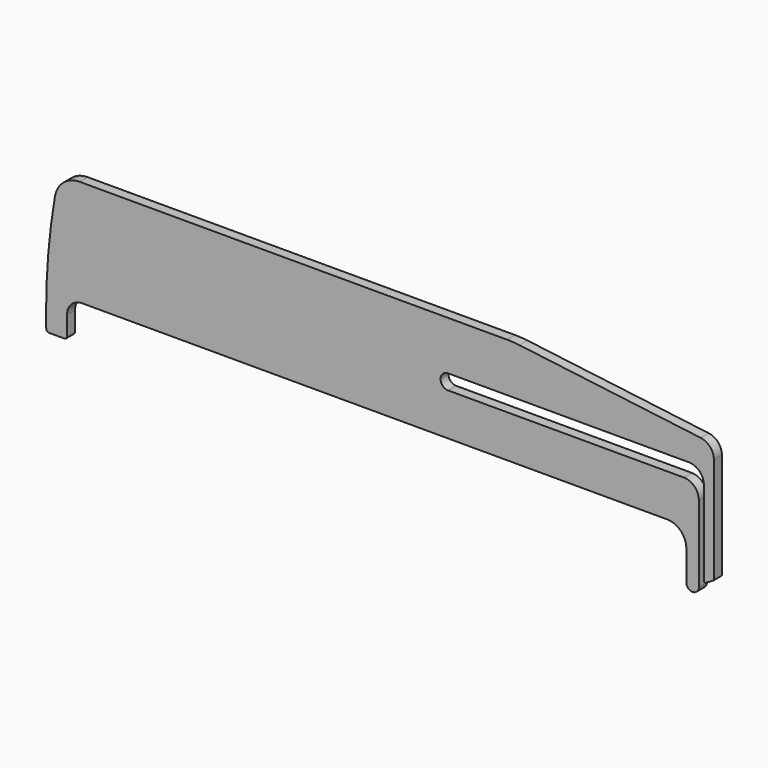
from build123d import *

# Parameters (mm, degrees)
F1_DEPTH = 1


# Not quite as in the source:
# - a feature names something its author has since deleted; it is built from what else it names


with BuildPart() as f1:
    # F0 (on Front) → F1 (new body, symmetric)
    with BuildSketch(Plane.XZ):
        with BuildLine():
            ThreePointArc((-58.215127866, 20.8417536759), (-59.5395660257, 10.4582609311), (-59.9821, 0))
            ThreePointArc((-59.9821, 0), (-59.9729371877, -1.5061942231), (-59.9454501071, -3.0121654896))
            ThreePointArc((-59.9454501071, -3.0121654896), (-59.7948238827, -3.3578286914), (-59.4455981282, -3.5))
            Line((-59.4455981282, -3.5), (-56.3175, -3.5))
            ThreePointArc((-56.3175, -3.5), (-55.9639466094, -3.3535533906), (-55.8175, -3))
            Line((-55.8175, -3), (-55.8175, 0.8354))
            ThreePointArc((-55.8175, 0.8354), (-54.9388203436, 2.9567203436), (-52.8175, 3.8354))
            Line((-52.8175, 3.8354), (63.8175, 3.8354))
            ThreePointArc((63.8175, 3.8354), (66.5295373486, 2.7120373486), (67.6529, 0))
            Line((67.6529, 0), (67.6529, -6))
            ThreePointArc((67.6529, -6), (68.9029, -7.25), (70.1529, -6))
            Line((70.1529, -6), (70.1529, 9.2687909752))
            ThreePointArc((70.1529, 9.2687909752), (69.2742203436, 11.3901113188), (67.1529, 12.2687909752))
            Line((67.1529, 12.2687909752), (20.1529, 12.2687909752))
            ThreePointArc((20.1529, 12.2687909752), (18.6529, 13.7687909752), (20.1529, 15.2687909752))
            Line((20.1529, 15.2687909752), (68.1529, 15.2687909752))
            ThreePointArc((68.1529, 15.2687909752), (70.2742203436, 14.3901113188), (71.1529, 12.2687909752))
            Line((71.1529, 12.2687909752), (71.1529, -4.5669872981))
            ThreePointArc((71.1529, -4.5669872981), (71.2779, -4.7834936491), (71.5279, -4.7834936491))
            Line((71.5279, -4.7834936491), (73.0279, -3.9174682453))
            ThreePointArc((73.0279, -3.9174682453), (73.1194063509, -3.8259618943), (73.1529, -3.7009618943))
            Line((73.1529, -3.7009618943), (73.1529, 17.3516533444))
            ThreePointArc((73.1529, 17.3516533444), (72.4019345274, 19.3370610341), (70.5250042038, 20.3284869745))
            Line((70.5250042038, 20.3284869745), (34.3884397258, 24.8455575343))
            ThreePointArc((34.3884397258, 24.8455575343), (33.1504938652, 24.961352042), (31.907745034, 25))
            Line((31.907745034, 25), (-53.2864920761, 25))
            ThreePointArc((-53.2864920761, 25), (-56.510715364, 23.8215682893), (-58.215127866, 20.8417536759))
        make_face()
    extrude(amount=F1_DEPTH, both=True)


solid = f1.part
